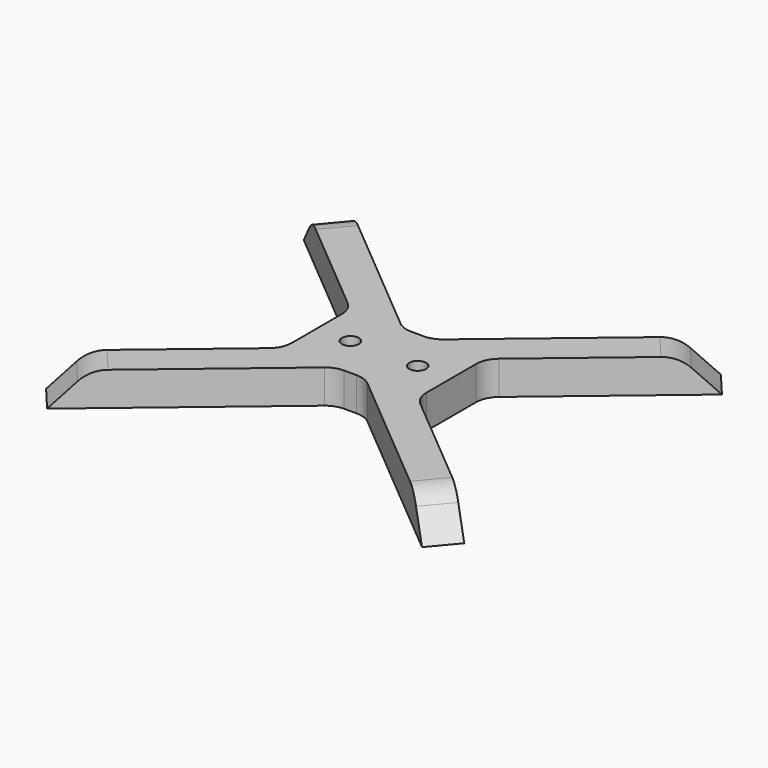
from build123d import *

# Parameters (mm, degrees)
F0_R     = 5
F0_R_2   = 2.5
F1_DEPTH = 10
F2_DEPTH = 5
F3_SIZE  = 9.99999
F4_R     = 7
F5_R     = 10


# Not quite as in the source:
# - a fillet or chamfer is up to 0.001 mm smaller than in the source, because OpenCascade refuses the exact size


with BuildPart() as f1:
    # F0 (on Top) → F1 (new body)
    with BuildSketch(Plane.XY):
        Polygon((4.4427617314, -12.5), (20, -12.5), (20, 12.5), (4.4427617314, 12.5), (-4.4427617314, 12.5), (-20, 12.5), (-20, -12.5), (-4.4427617314, -12.5), align=None)
        with Locations((-10, 0)):
            Circle(F0_R, mode=Mode.SUBTRACT)
        with Locations((10, 0)):
            Circle(F0_R, mode=Mode.SUBTRACT)
        Polygon((-55.7045682747, -55.5137629639), (-4.4427617314, -12.5), (-20, -12.5), (-62.1324443715, -47.8533185328), align=None)
        Polygon((62.1324443715, -47.8533185328), (20, -12.5), (4.4427617314, -12.5), (55.7045682747, -55.5137629639), align=None)
        Polygon((4.4427617314, 12.5), (20, 12.5), (62.1324443715, 47.8533185328), (55.7045682747, 55.5137629639), align=None)
        Polygon((-20, 12.5), (-4.4427617314, 12.5), (-55.7045682747, 55.5137629639), (-62.1324443715, 47.8533185328), align=None)
        with Locations((10, 0)):
            Circle(F0_R)
        with Locations((10, 0)):
            Circle(F0_R_2, mode=Mode.SUBTRACT)
        with Locations((-10, 0)):
            Circle(F0_R)
        with Locations((-10, 0)):
            Circle(F0_R_2, mode=Mode.SUBTRACT)
    extrude(amount=F1_DEPTH)

    # F0 (on Top) → F2 (cut)
    with BuildSketch(Plane.XY):
        with Locations((-10, 0)):
            Circle(F0_R)
        with Locations((-10, 0)):
            Circle(F0_R_2, mode=Mode.SUBTRACT)
        with Locations((10, 0)):
            Circle(F0_R)
        with Locations((10, 0)):
            Circle(F0_R_2, mode=Mode.SUBTRACT)
    extrude(amount=F2_DEPTH, mode=Mode.SUBTRACT)

    # F3 (size 10 in the source; OpenCascade refuses exactly that, so slightly less here)
    f3_edges = [f1.edges().sort_by_distance(p)[0] for p in [
        (58.918506, -51.683541, 10),
        (58.918506, 51.683541, 10),
        (-58.918506, 51.683541, 10),
        (-58.918506, -51.683541, 10),
    ]]
    chamfer(f3_edges, length=F3_SIZE)

    # F4
    f4_edges = [f1.edges().sort_by_distance(p)[0] for p in [
        (4.442762, 12.5, 5),
        (-4.442762, 12.5, 5),
        (4.442762, -12.5, 5),
        (-4.442762, -12.5, 5),
        (-20, -12.5, 5),
        (-20, 12.5, 5),
        (20, -12.5, 5),
        (20, 12.5, 5),
    ]]
    fillet(f4_edges, radius=F4_R)

    # F5
    f5_edges = [f1.edges().sort_by_distance(p)[0] for p in [
        (-51.25807, 45.255671, 10),
        (-51.25807, -45.255671, 10),
        (51.25807, 45.255671, 10),
        (51.25807, -45.255671, 10),
    ]]
    fillet(f5_edges, radius=F5_R)


solid = f1.part
